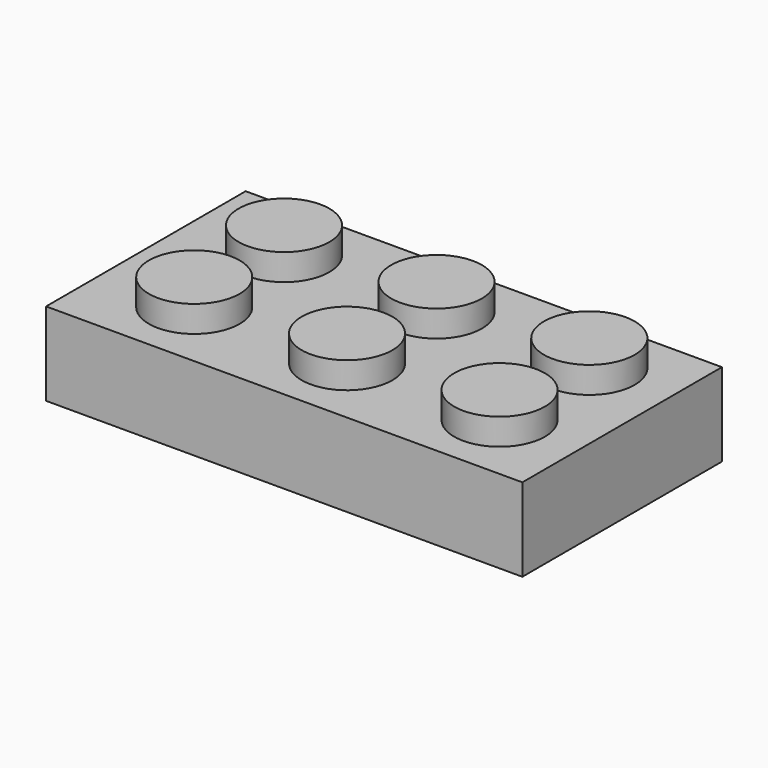
from build123d import *

# Parameters (mm, degrees)
F0_W     = 126
F0_H     = 66
F0_W_2   = 120
F0_H_2   = 60
F1_DEPTH = 21
F2_W     = 126
F2_H     = 66
F3_DEPTH = 1
F0_R     = 12
F4_DEPTH = 8
F6_DEPTH = 22


with BuildPart() as f1:
    # F0 (on Top) → F1 (new body)
    with BuildSketch(Plane.XY):
        with Locations((-1.5, -1.5)):
            Rectangle(F0_W, F0_H)
        with Locations((-1.5, -1.5)):
            Rectangle(F0_W_2, F0_H_2, mode=Mode.SUBTRACT)
    extrude(amount=-F1_DEPTH)

    # F2 (on face) → F3 (join)
    with BuildSketch(Plane.XY):
        with Locations((-1.5, -1.5)):
            Rectangle(F2_W, F2_H)
    extrude(amount=F3_DEPTH)

    # F0 (on Top) → F4 (join)
    with BuildSketch(Plane.XY):
        with Locations((-40.3844975889, 14.0422494113)):
            Circle(F0_R)
        with Locations((0, 14)):
            Circle(F0_R)
        with Locations((-40.3844975889, -15.6422494113)):
            Circle(F0_R)
        with Locations((0, -15.6)):
            Circle(F0_R)
        with Locations((40.3844975889, -15.6422494113)):
            Circle(F0_R)
        with Locations((40.3844975889, 14.0422494113)):
            Circle(F0_R)
    extrude(amount=F4_DEPTH)

    # F5 (on face) → F6 (join)
    with BuildSketch(Plane.XY):
        with BuildLine():
            ThreePointArc((31.4784805761, 5.99968384), (32.8922690999, 2.7143222033), (33.3752768321, -0.8295602165))
            ThreePointArc((33.3752768321, -0.8295602165), (32.9180007232, -4.2794585958), (31.5777529034, -7.4910993057))
            ThreePointArc((31.5777529034, -7.4910993057), (33.0771463209, -6.123708691), (34.7855065256, -5.0285177832))
            ThreePointArc((34.7855065256, -5.0285177832), (35.2271141548, -2.9496471052), (35.3752768321, -0.8295602165))
            ThreePointArc((35.3752768321, -0.8295602165), (35.2220188743, 1.3264920966), (34.7653269231, 3.4391875409))
            ThreePointArc((34.7653269231, 3.4391875409), (33.0099261031, 4.57569273), (31.4784805761, 5.99968384))
        make_face()
        with BuildLine():
            ThreePointArc((30.044931449, 7.9518165828), (30.8064288175, 7.0085924135), (31.4784805761, 5.99968384))
            ThreePointArc((31.4784805761, 5.99968384), (33.0099261031, 4.57569273), (34.7653269231, 3.4391875409))
            ThreePointArc((34.7653269231, 3.4391875409), (32.4184567267, 8.1923854782), (28.5856333111, 11.8543733283))
            ThreePointArc((28.5856333111, 11.8543733283), (29.1446126861, 9.8392757768), (30.044931449, 7.9518165828))
        make_face()
        with BuildLine():
            ThreePointArc((34.7855065256, -5.0285177832), (33.0771463209, -6.123708691), (31.5777529034, -7.4910993057))
            ThreePointArc((31.5777529034, -7.4910993057), (30.8212956484, -8.6474276201), (29.948463719, -9.718635897))
            ThreePointArc((29.948463719, -9.718635897), (29.0995516946, -11.5618087289), (28.5733528944, -13.5216690648))
            ThreePointArc((28.5733528944, -13.5216690648), (32.4355688891, -9.8281570151), (34.7855065256, -5.0285177832))
        make_face()
        with BuildLine():
            ThreePointArc((10.5845976874, 8.3461259481), (20.4011056558, 12.410159384), (30.044931449, 7.9518165828))
            ThreePointArc((30.044931449, 7.9518165828), (29.1446126861, 9.8392757768), (28.5856333111, 11.8543733283))
            ThreePointArc((28.5856333111, 11.8543733283), (20.2186418923, 14.4126354365), (11.8233794228, 11.9487323369))
            ThreePointArc((11.8233794228, 11.9487323369), (11.3478655588, 10.0979560153), (10.5845976874, 8.3461259481))
        make_face()
        with BuildLine():
            ThreePointArc((28.5733528944, -13.5216690648), (29.0995516946, -11.5618087289), (29.948463719, -9.718635897))
            ThreePointArc((29.948463719, -9.718635897), (20.3778358891, -14.0697308571), (10.652789482, -10.0756831869))
            ThreePointArc((10.652789482, -10.0756831869), (11.3821848264, -11.7992278973), (11.8347224415, -13.615221742))
            ThreePointArc((11.8347224415, -13.615221742), (20.2180287599, -16.0717593087), (28.5733528944, -13.5216690648))
        make_face()
        with BuildLine():
            ThreePointArc((8.5383868776, 5.5681585921), (9.4706325231, 7.0240682624), (10.5845976874, 8.3461259481))
            ThreePointArc((10.5845976874, 8.3461259481), (11.3478655588, 10.0979560153), (11.8233794228, 11.9487323369))
            ThreePointArc((11.8233794228, 11.9487323369), (7.86032363, 8.2101986383), (5.4651898622, 3.3167561214))
            ThreePointArc((5.4651898622, 3.3167561214), (7.0917024506, 4.3197233329), (8.5383868776, 5.5681585921))
        make_face()
        with BuildLine():
            ThreePointArc((11.8347224415, -13.615221742), (11.3821848264, -11.7992278973), (10.652789482, -10.0756831869))
            ThreePointArc((10.652789482, -10.0756831869), (9.455680238, -8.6628486697), (8.46736073, -7.0968357497))
            ThreePointArc((8.46736073, -7.0968357497), (7.0422594659, -5.8836950637), (5.4458638506, -4.9068916156))
            ThreePointArc((5.4458638506, -4.9068916156), (7.8431131072, -9.8459070996), (11.8347224415, -13.615221742))
        make_face()
        with BuildLine():
            ThreePointArc((8.46736073, -7.0968357497), (6.8906107626, -0.7552968983), (8.5383868776, 5.5681585921))
            ThreePointArc((8.5383868776, 5.5681585921), (7.0917024506, 4.3197233329), (5.4651898622, 3.3167561214))
            ThreePointArc((5.4651898622, 3.3167561214), (4.8904446173, -0.7937397736), (5.4458638506, -4.9068916156))
            ThreePointArc((5.4458638506, -4.9068916156), (7.0422594659, -5.8836950637), (8.46736073, -7.0968357497))
        make_face()
        with BuildLine():
            ThreePointArc((-8.5383868776, 5.5681585921), (-7.0917024506, 4.3197233329), (-5.4651898622, 3.3167561214))
            ThreePointArc((-5.4651898622, 3.3167561214), (-7.86032363, 8.2101986383), (-11.8233794228, 11.9487323369))
            ThreePointArc((-11.8233794228, 11.9487323369), (-11.3478655588, 10.0979560153), (-10.5845976874, 8.3461259481))
            ThreePointArc((-10.5845976874, 8.3461259481), (-9.4706325231, 7.0240682624), (-8.5383868776, 5.5681585921))
        make_face()
        with BuildLine():
            ThreePointArc((-4.8904025274, -0.8295602165), (-5.034783168, 1.2634232792), (-5.4651898622, 3.3167561214))
            ThreePointArc((-5.4651898622, 3.3167561214), (-7.0917024506, 4.3197233329), (-8.5383868776, 5.5681585921))
            ThreePointArc((-8.5383868776, 5.5681585921), (-7.3090150887, 2.4737206667), (-6.8904025274, -0.8295602165))
            ThreePointArc((-6.8904025274, -0.8295602165), (-7.2906920093, -4.0608734086), (-8.46736073, -7.0968357497))
            ThreePointArc((-8.46736073, -7.0968357497), (-7.0422594659, -5.8836950637), (-5.4458638506, -4.9068916156))
            ThreePointArc((-5.4458638506, -4.9068916156), (-5.0299062498, -2.8870567912), (-4.8904025274, -0.8295602165))
        make_face()
        with BuildLine():
            ThreePointArc((-10.5845976874, 8.3461259481), (-11.3478655588, 10.0979560153), (-11.8233794228, 11.9487323369))
            ThreePointArc((-11.8233794228, 11.9487323369), (-20.2186418923, 14.4126354365), (-28.5856333111, 11.8543733283))
            ThreePointArc((-28.5856333111, 11.8543733283), (-29.1446126861, 9.8392757768), (-30.044931449, 7.9518165828))
            ThreePointArc((-30.044931449, 7.9518165828), (-20.4011056558, 12.410159384), (-10.5845976874, 8.3461259481))
        make_face()
        with BuildLine():
            ThreePointArc((-11.8347224415, -13.615221742), (-7.8431131072, -9.8459070996), (-5.4458638506, -4.9068916156))
            ThreePointArc((-5.4458638506, -4.9068916156), (-7.0422594659, -5.8836950637), (-8.46736073, -7.0968357497))
            ThreePointArc((-8.46736073, -7.0968357497), (-9.455680238, -8.6628486697), (-10.652789482, -10.0756831869))
            ThreePointArc((-10.652789482, -10.0756831869), (-11.3821848264, -11.7992278973), (-11.8347224415, -13.615221742))
        make_face()
        with BuildLine():
            ThreePointArc((-28.5733528944, -13.5216690648), (-20.2180287599, -16.0717593087), (-11.8347224415, -13.615221742))
            ThreePointArc((-11.8347224415, -13.615221742), (-11.3821848264, -11.7992278973), (-10.652789482, -10.0756831869))
            ThreePointArc((-10.652789482, -10.0756831869), (-20.3778358891, -14.0697308571), (-29.948463719, -9.718635897))
            ThreePointArc((-29.948463719, -9.718635897), (-29.0995516946, -11.5618087289), (-28.5733528944, -13.5216690648))
        make_face()
        with BuildLine():
            ThreePointArc((-30.044931449, 7.9518165828), (-29.1446126861, 9.8392757768), (-28.5856333111, 11.8543733283))
            ThreePointArc((-28.5856333111, 11.8543733283), (-32.4184567267, 8.1923854782), (-34.7653269231, 3.4391875409))
            ThreePointArc((-34.7653269231, 3.4391875409), (-33.0099261031, 4.57569273), (-31.4784805761, 5.99968384))
            ThreePointArc((-31.4784805761, 5.99968384), (-30.8064288175, 7.0085924135), (-30.044931449, 7.9518165828))
        make_face()
        with BuildLine():
            ThreePointArc((-34.7855065256, -5.0285177832), (-32.4355688891, -9.8281570151), (-28.5733528944, -13.5216690648))
            ThreePointArc((-28.5733528944, -13.5216690648), (-29.0995516946, -11.5618087289), (-29.948463719, -9.718635897))
            ThreePointArc((-29.948463719, -9.718635897), (-30.8212956484, -8.6474276201), (-31.5777529034, -7.4910993057))
            ThreePointArc((-31.5777529034, -7.4910993057), (-33.0771463209, -6.123708691), (-34.7855065256, -5.0285177832))
        make_face()
        with BuildLine():
            ThreePointArc((-31.4784805761, 5.99968384), (-33.0099261031, 4.57569273), (-34.7653269231, 3.4391875409))
            ThreePointArc((-34.7653269231, 3.4391875409), (-35.3752335492, -0.7932356825), (-34.7855065256, -5.0285177832))
            ThreePointArc((-34.7855065256, -5.0285177832), (-33.0771463209, -6.123708691), (-31.5777529034, -7.4910993057))
            ThreePointArc((-31.5777529034, -7.4910993057), (-33.3749183212, -0.7321179887), (-31.4784805761, 5.99968384))
        make_face()
    extrude(amount=-F6_DEPTH)


solid = f1.part
